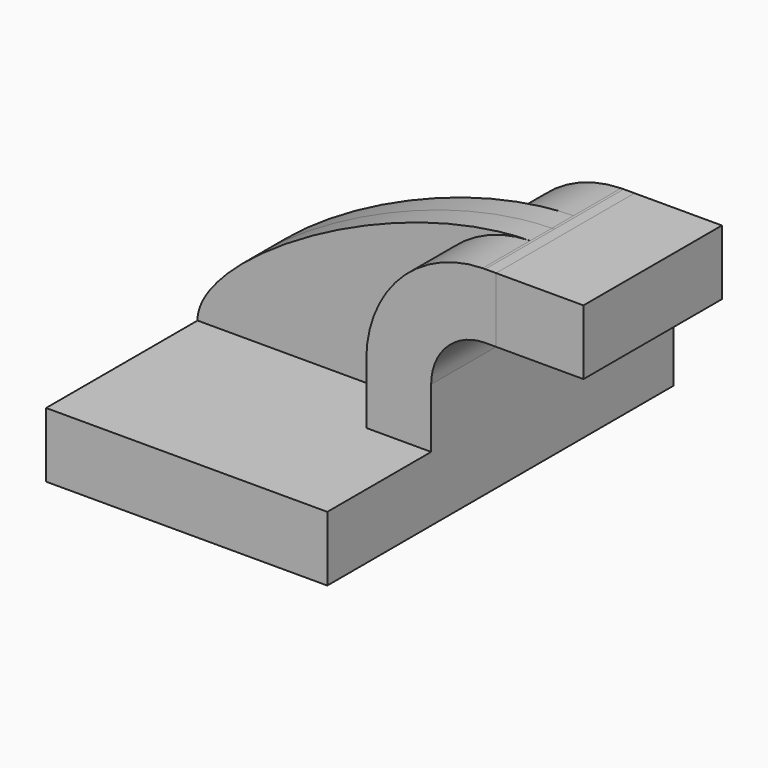
from build123d import *

# Parameters (mm, degrees)
F1_DEPTH = 63.5
F2_DEPTH = 25.4
F3_DEPTH = 7.9375
F4_DEPTH = 25.4


# Not quite as in the source:
# - a feature of the source that left no trace in its solid (it failed there, or was rolled back) is left out


with BuildPart() as f1:
    # F0 (on Front) → F1 (new body, symmetric)
    with BuildSketch(Plane.XZ):
        Polygon((-41.275, -9.525), (41.275, -9.525), (41.275, 9.525), (22.225, 9.525), (-41.275, 9.525), align=None)
    extrude(amount=F1_DEPTH, both=True)

    # F0 (on Front) → F2 (join, symmetric)
    with BuildSketch(Plane.XZ):
        with BuildLine():
            Line((22.225, 9.525), (41.275, 9.525))
            Line((41.275, 9.525), (41.275, 27.0002))
            ThreePointArc((41.275, 27.0002), (45.9246798487, 38.2255201513), (57.15, 42.8752))
            Line((57.15, 42.8752), (60.325, 42.8752))
            Line((60.325, 42.8752), (60.325, 61.9252))
            Line((60.325, 61.9252), (57.15, 61.9252))
            add(Edge.make_bspline(
                [(56.3910941137, 61.9169536701), (56.6445667291, 61.920927039), (56.8975404447, 61.9236794966), (57.15, 61.9252)],
                knots=[110.8367961001, 110.8367961001, 110.8367961001, 110.8367961001, 111.5045361635, 111.5045361635, 111.5045361635, 111.5045361635], degree=3))
            ThreePointArc((56.3910941137, 61.9169536701), (32.1874238801, 51.4261169421), (22.225, 27.0002))
            Line((22.225, 27.0002), (22.225, 9.525))
        make_face()
    extrude(amount=F2_DEPTH, both=True)

    # F0 (on Front) → F3 (join, symmetric)
    with BuildSketch(Plane.XZ):
        with BuildLine():
            add(Edge.make_bspline(
                [(-41.275, 9.525), (-41.5013838276, 26.9593473463), (14.3176973965, 61.2574223543), (56.3910941137, 61.9169536701)],
                knots=[0, 0, 0, 0, 110.8367961001, 110.8367961001, 110.8367961001, 110.8367961001], degree=3))
            Line((-41.275, 9.525), (22.225, 9.525))
            Line((22.225, 9.525), (22.225, 27.0002))
            ThreePointArc((22.225, 27.0002), (32.1874238801, 51.4261169421), (56.3910941137, 61.9169536701))
        make_face()
    extrude(amount=F3_DEPTH, both=True)


with BuildPart() as f2:
    # F0 (on Front) → F2, piece 2 (new body, symmetric)
    with BuildSketch(Plane.XZ):
        Polygon((85.7910350956, 61.9252), (85.8969844585, 42.8752), (85.9816285353, 42.8752), (85.9816285353, 61.9252), align=None)
    extrude(amount=F2_DEPTH, both=True)


with BuildPart() as f4:
    # F0 (on Front) → F4 (new body, symmetric)
    with BuildSketch(Plane.XZ):
        Polygon((60.325, 61.9252), (60.325, 42.8752), (85.8969844585, 42.8752), (85.7910350956, 61.9252), align=None)
    extrude(amount=F4_DEPTH, both=True)


solid = Compound([f1.part, f2.part, f4.part])
